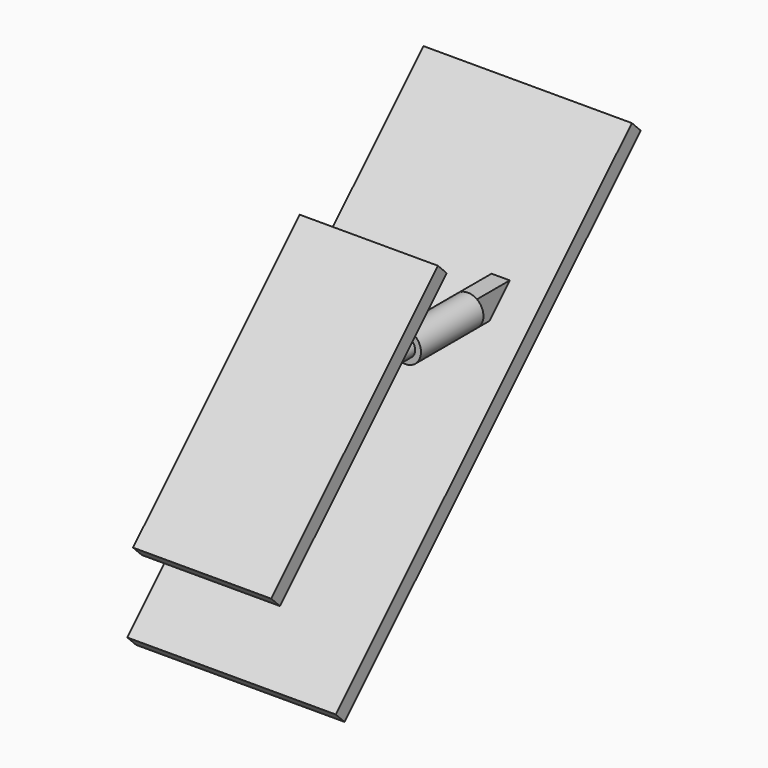
from build123d import *

# Parameters (mm, degrees)
F0_R         = 25.4
F1_DEPTH     = 127
F2_R         = 15.875
F3_DEPTH     = 203.2
F4_W         = 18.542
F4_H         = 25.7731786165
F5_DEPTH     = 25.4
F6_SIZE      = 25.39999
F7_W         = 18.542
F7_H         = 35.9210244843
F8_DEPTH     = 12.7
F9_W         = 29.620467016
F9_H         = 41.2706667472
F10_DEPTH    = 76.2
F11_T1_DEPTH = 290.9034585933
F12_W        = 224.6891856194
F12_H        = 479.333948344
F13_DEPTH    = 25.4
F14_W        = 338.9952555299
F14_H        = 851.445376873
F15_DEPTH    = 25.4


# Not quite as in the source:
# - a fillet or chamfer that OpenCascade refuses, or shapes differently, is made with other operations: its cross-section is extruded or revolved along the edge and cut away or added
# - a fillet or chamfer is up to 0.001 mm smaller than in the source, because OpenCascade refuses the exact size


with BuildPart() as f1:
    # F0 (on Front) → F1 (new body)
    with BuildSketch(Plane.XZ):
        Circle(F0_R)
    extrude(amount=F1_DEPTH)

    # F2 (on face) → F3 (join)
    with BuildSketch(Plane.XZ.offset(127)):
        Circle(F2_R)
    extrude(amount=F3_DEPTH)

    # F4 (on face) → F5 (join)
    with BuildSketch(Plane.XZ.offset(330.2)):
        Rectangle(F4_W, F4_H)
    extrude(amount=F5_DEPTH)

    # F6 (size 25.4 in the source; OpenCascade refuses exactly that, so slightly less here)
    f6_edges = [f1.edges().sort_by_distance(p)[0] for p in [
        (0, -355.6, 12.886589),
    ]]
    chamfer(f6_edges, length=F6_SIZE)

    # F7 (on face) → F8 (join)
    with BuildSketch(Plane(origin=(0, -171.5432946541, 171.5432946541), x_dir=(1, 0, 0), z_dir=(0, -0.7071067812, 0.7071067812))):
        with Locations((0, -242.3349767037)):
            Rectangle(F7_W, F7_H)
    extrude(amount=F8_DEPTH)

    # F9 (on face) → F10 (join)
    with BuildSketch(Plane(origin=(0, 0, 0), x_dir=(-1, 0, 0), z_dir=(0, 1, 0))):
        with Locations((-1.508e-06, -1.0823e-06)):
            Rectangle(F9_W, F9_H)
    extrude(amount=F10_DEPTH)

    # F11: chamfer of 50.8 on 1 edges, made by hand

    # F11_s2 → F11_t1 (cut)
    with BuildSketch(Plane.YZ.offset(-145.4517277887)):
        Polygon((25.4, -20.6353344559), (76.2, 30.1646655441), (76.2, -20.6353344559), align=None)
    extrude(amount=F11_T1_DEPTH, mode=Mode.SUBTRACT)

    # F12 (on face) → F13 (join)
    with BuildSketch(Plane(origin=(0, -180.5235507752, 180.5235507752), x_dir=(1, 0, 0), z_dir=(0, -0.7071067812, 0.7071067812))):
        with Locations((6.4224079251, -255.024516955)):
            Rectangle(F12_W, F12_H)
    extrude(amount=F13_DEPTH)

    # F14 (on face) → F15 (join)
    with BuildSketch(Plane(origin=(0, 23.0176672279, -23.0176672279), x_dir=(1, 0, 0), z_dir=(0, 0.7071067812, -0.7071067812))):
        with Locations((-95.1869599521, 118.0603802204)):
            Rectangle(F14_W, F14_H)
    extrude(amount=F15_DEPTH)


solid = f1.part
